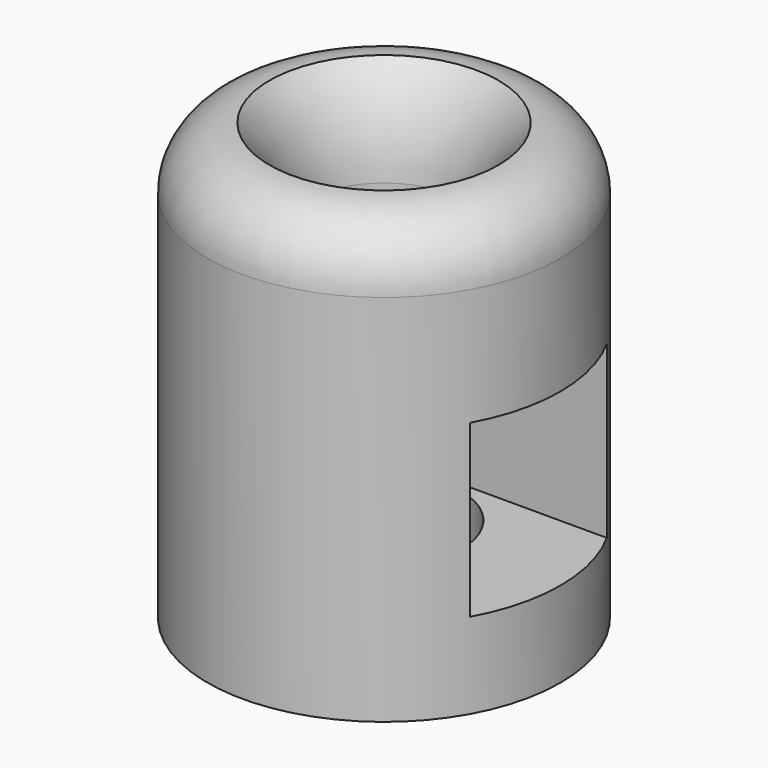
from build123d import *

# Parameters (mm, degrees)
F0_R     = 38.5018988787
F0_R_2   = 16.939934048
F1_DEPTH = 95
F5_W     = 37.283
F5_H     = 37.253003633
F6_DEPTH = 100
F7_R     = 13.5195959493


# Not quite as in the source:
# - a fillet or chamfer that OpenCascade refuses, or shapes differently, is made with other operations: its cross-section is extruded or revolved along the edge and cut away or added


with BuildPart() as f1:
    # F0 (on Top) → F1 (new body)
    with BuildSketch(Plane.XY):
        Circle(F0_R)
        Circle(F0_R_2, mode=Mode.SUBTRACT)
    extrude(amount=F1_DEPTH)

    # F5 (on line) → F6 (cut)
    with BuildSketch(Plane.YZ.offset(-38.5018988787)):
        with Locations((0, 37.3)):
            Rectangle(F5_W, F5_H)
    extrude(amount=F6_DEPTH, mode=Mode.SUBTRACT)

    # F7
    f7_edges = [f1.edges().sort_by_distance(p)[0] for p in [
        (-38.501899, 0, 95),
    ]]
    fillet(f7_edges, radius=F7_R)

    # F8: fillet of radius 29.8468724241 on 1 edges, made by hand

    # F8_s1 → F8_t2 (revolve, cut)
    with BuildSketch(Plane.XZ):
        with BuildLine():
            ThreePointArc((24.9823029294, 95), (19.0232329538, 85.5740041188), (16.939934048, 74.6186502225))
            Line((16.939934048, 74.6186502225), (16.939934048, 95))
            Line((16.939934048, 95), (24.9823029294, 95))
        make_face()
    revolve(axis=Axis((0, 0, 95), (0, 0, 1)), mode=Mode.SUBTRACT)


solid = f1.part
